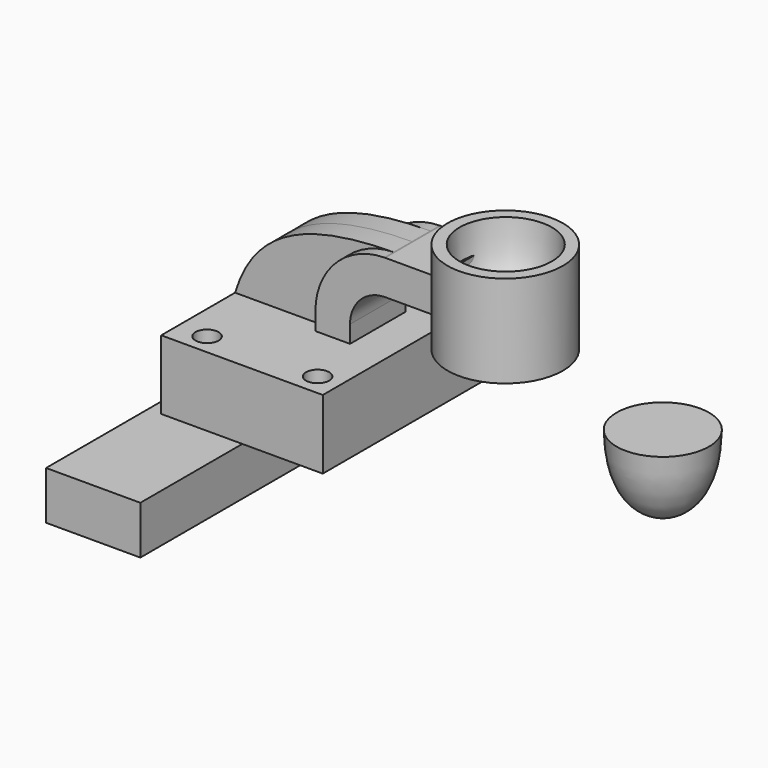
from build123d import *

# Parameters (mm, degrees)
F1_DEPTH  = 63.5
F2_DEPTH  = 12.7
F0_W      = 31.75
F0_H      = 50.8
F4_DEPTH  = 19.05
F8_R      = 6.35
F9_DEPTH  = 38.1
F11_W     = 51.8660424277
F11_H     = 26.5504792333
F12_DEPTH = 116.078


# Not quite as in the source:
# - ends of sketch curves that miss each other by under 0.0002 mm in the source are joined


with BuildPart() as f1:
    # F0 (on Front) → F1 (new body, symmetric)
    with BuildSketch(Plane.XZ):
        Polygon((7.7104573138, 24.8640864372), (-41.5579093681, 24.8640864372), (-41.5579093681, -13.2359135628), (47.3420906319, -13.2359135628), (47.3420906319, 24.8640864372), (26.7604570836, 24.8640864372), align=None)
    extrude(amount=F1_DEPTH, both=True)

    # F0 (on Front) → F2 (join, symmetric)
    with BuildSketch(Plane.XZ):
        with BuildLine():
            add(Edge.make_bspline(
                [(-41.5579093681, 24.8640864372), (-31.1663596882, 59.2701950139), (-3.3499980814, 72.437082025), (45.6389581324, 72.8365695774)],
                knots=[0, 0, 0, 0, 99.6343082165, 99.6343082165, 99.6343082165, 99.6343082165], degree=3))
            Line((-41.5579093681, 24.8640864372), (7.7104573138, 24.8640864372))
            Line((7.7104573138, 24.8640864372), (7.7104573138, 34.3604520069))
            ThreePointArc((7.7104573138, 34.3604520069), (18.7866933694, 61.3742578065), (45.6389581324, 72.8365695774))
        make_face()
    extrude(amount=F2_DEPTH, both=True)


with BuildPart() as f3:
    # F0 (on Front) → F3 (revolve)
    with BuildSketch(Plane.XZ):
        with Locations((112.7920650244, 62.6620671988)):
            Rectangle(F0_W, F0_H)
    revolve(axis=Axis((96.9170650244, 0, 62.6620671988), (0, 0, -1)))


with BuildPart() as f4:
    # F0 (on Front) → F4 (new body, symmetric)
    with BuildSketch(Plane.XZ):
        with BuildLine():
            Line((7.7104573138, 34.3604520069), (7.7104573138, 24.8640864372))
            Line((7.7104573138, 24.8640864372), (26.7604570836, 24.8640864372))
            Line((26.7604570836, 24.8640864372), (26.7604570836, 34.3604520069))
            ThreePointArc((26.7604570836, 34.3604520069), (32.4513930763, 48.0995868632), (46.1905279326, 53.7905228559))
            Line((46.1905279326, 53.7905228559), (74.5775754276, 53.7905228559))
            Line((74.5775754276, 53.7905228559), (74.5775754276, 72.8405192494))
            Line((74.5775754276, 72.8405192494), (46.1905279326, 72.8405192494))
            add(Edge.make_bspline(
                [(45.6389581324, 72.8365695774), (45.8225174109, 72.8380664382), (46.0063739453, 72.8393840491), (46.1905279326, 72.8405192494)],
                knots=[99.6343082165, 99.6343082165, 99.6343082165, 99.6343082165, 100.0076332094, 100.0076332094, 100.0076332094, 100.0076332094], degree=3))
            ThreePointArc((45.6389581324, 72.8365695774), (18.7866933694, 61.3742578065), (7.7104573138, 34.3604520069))
        make_face()
    extrude(amount=F4_DEPTH, both=True)


with BuildPart() as f5:
    # F0 (on Front) → F5 (revolve)
    with BuildSketch(Plane.XZ):
        with BuildLine():
            Line((183.6182943821, 26.596263051), (158.2182943821, 26.596263051))
            add(Edge.make_bspline(
                [(158.2182943821, 26.596263051), (158.61569345, 0), (168.516787076, -12.7471527085), (183.6182943821, -14.3367853016)],
                knots=[0, 0, 0, 0, 48.1733790328, 48.1733790328, 48.1733790328, 48.1733790328], degree=3))
            Line((183.6182943821, -14.3367853016), (183.6182943821, 26.596263051))
        make_face()
    revolve(axis=Axis((183.6182943821, 0, 6.1297388747), (0, 0, 1)))


with BuildPart() as f6_1:
    # F6: copy of F5
    add(f5.part.moved(Location((-86.614, 0.254, 62.992))))


with BuildPart() as f3_1:
    add(f3.part)

    # F7: cut F6_1
    add(f6_1.part, mode=Mode.SUBTRACT)


with BuildPart() as f9:
    # F8 (on Top) → F9 (new body, symmetric)
    with BuildSketch(Plane.XY):
        with Locations((-26.8744081259, 49.222741276)):
            Circle(F8_R)
    extrude(amount=F9_DEPTH, both=True)


with BuildPart() as f9b:
    # F8 (on Top) → F9, piece 2 (new body, symmetric)
    with BuildSketch(Plane.XY):
        with Locations((33.5120453119, 49.7758090496)):
            Circle(F8_R)
    extrude(amount=F9_DEPTH, both=True)


with BuildPart() as f9c:
    # F8 (on Top) → F9, piece 3 (new body, symmetric)
    with BuildSketch(Plane.XY):
        with Locations((-25.5839244187, -51.9409514964)):
            Circle(F8_R)
    extrude(amount=F9_DEPTH, both=True)


with BuildPart() as f9d:
    # F8 (on Top) → F9, piece 4 (new body, symmetric)
    with BuildSketch(Plane.XY):
        with Locations((34.8025290191, -51.3878837228)):
            Circle(F8_R)
    extrude(amount=F9_DEPTH, both=True)


with BuildPart() as f1_1:
    add(f1.part)

    # F10: cut F9c, F9d, F9, F9b
    add(f9c.part, mode=Mode.SUBTRACT)
    add(f9d.part, mode=Mode.SUBTRACT)
    add(f9.part, mode=Mode.SUBTRACT)
    add(f9b.part, mode=Mode.SUBTRACT)


with BuildPart() as f12:
    # F11 (on Front) → F12 (new body)
    with BuildSketch(Plane.XZ):
        with Locations((-36.9113073684, -38.2168479264)):
            Rectangle(F11_W, F11_H)
    extrude(amount=F12_DEPTH)


solid = Compound([f4.part, f5.part, f3_1.part, f1_1.part, f12.part])
